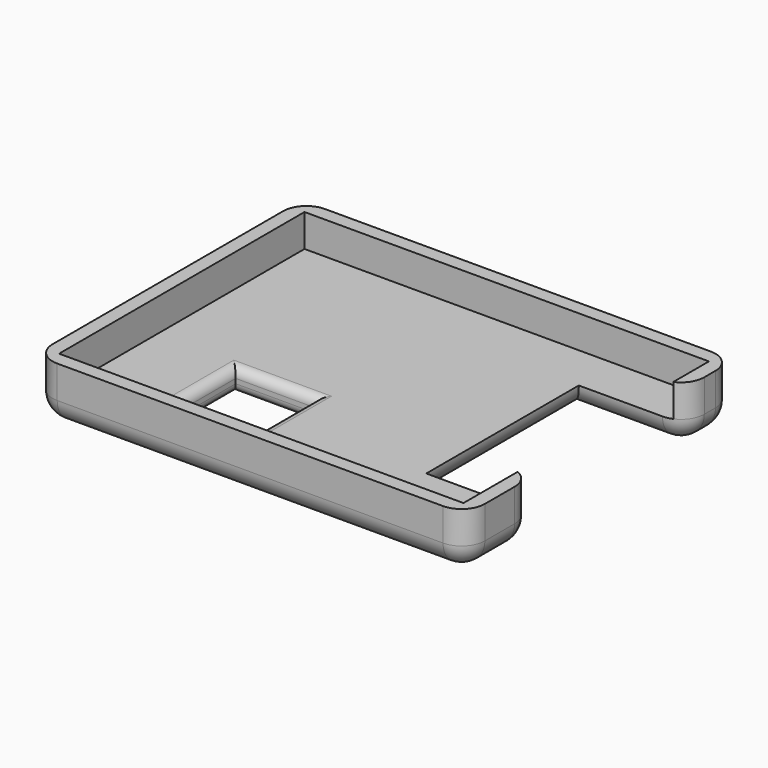
from build123d import *

# Parameters (mm, degrees)
F1_DEPTH = 12
F0_W     = 17
F0_H     = 20
F2_DEPTH = 5
F3_R     = 4.99999
F4_R     = 2


# Not quite as in the source:
# - a fillet or chamfer is up to 0.001 mm smaller than in the source, because OpenCascade refuses the exact size


with BuildPart() as f1:
    # F0 (on Top) → F1 (new body)
    with BuildSketch(Plane.XY):
        Polygon((-43.5, 33), (43.5, 33), (43.5, 23), (46.5, 23), (46.5, 36), (-46.5, 36), (-46.5, -36), (46.5, -36), (46.5, -18), (43.5, -18), (43.5, -33), (-43.5, -33), align=None)
    extrude(amount=F1_DEPTH)

    # F0 (on Top) → F2 (join)
    with BuildSketch(Plane.XY):
        Polygon((43.5, 23), (43.5, 33), (-43.5, 33), (-43.5, -33), (43.5, -33), (43.5, -18), (23.5, -18), (23.5, 23), align=None)
        with Locations((-17, -18)):
            Rectangle(F0_W, F0_H, mode=Mode.SUBTRACT)
    extrude(amount=F2_DEPTH)

    # F3 (radius 5 in the source; OpenCascade refuses exactly that, so slightly less here)
    f3_edges = [f1.edges().sort_by_distance(p)[0] for p in [
        (23.5, 2.5, 0),
        (35, -18, 0),
        (35, 23, 0),
        (46.5, 29.5, 0),
        (46.5, -27, 0),
        (0, -36, 0),
        (0, 36, 0),
        (-46.5, 0, 0),
        (-46.5, 36, 6),
        (46.5, 36, 6),
        (46.5, -36, 6),
        (-46.5, -36, 6),
        (46.5, -18, 6),
        (46.5, 23, 6),
    ]]
    fillet(f3_edges, radius=F3_R)

    # F4
    f4_edges = [f1.edges().sort_by_distance(p)[0] for p in [
        (-25.5, -18, 5),
        (-17, -28, 5),
        (-17, -8, 5),
        (-8.5, -18, 5),
        (-17, -8, 0),
        (-25.5, -18, 0),
        (-17, -28, 0),
        (-8.5, -18, 0),
    ]]
    fillet(f4_edges, radius=F4_R)


solid = f1.part
